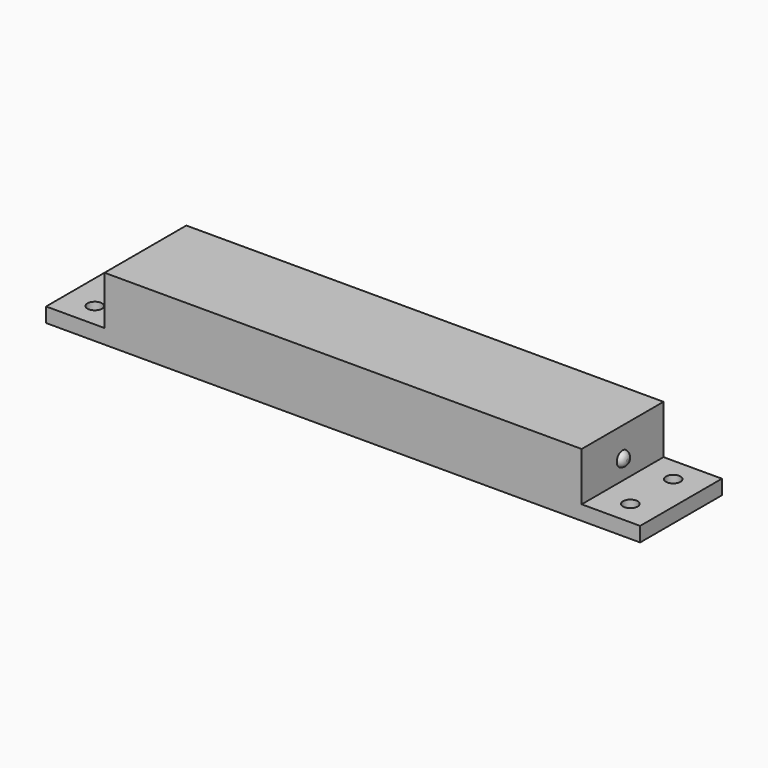
from build123d import *

# Parameters (mm, degrees)
F0_W     = 155.575
F0_H     = 33.3375
F1_DEPTH = 20.6375
F0_W_2   = 19.05
F0_R     = 2.38125
F2_DEPTH = 1.5875
F3_SIZE  = 1.27
F4_R     = 2.38125
F5_DEPTH = 1.5875
F7_DEPTH = 3.175


# Not quite as in the source:
# - a fillet or chamfer that OpenCascade refuses, or shapes differently, is made with other operations: its cross-section is extruded or revolved along the edge and cut away or added


with BuildPart() as f1:
    # F0 (on Top) → F1 (new body)
    with BuildSketch(Plane.XY):
        Rectangle(F0_W, F0_H)
    extrude(amount=F1_DEPTH)

    # F0 (on Top) → F2 (join)
    with BuildSketch(Plane.XY):
        with Locations((-87.3125, 0)):
            Rectangle(F0_W_2, F0_H)
        with Locations((-87.3125, -8.73125)):
            Circle(F0_R, mode=Mode.SUBTRACT)
        with Locations((-87.3125, 8.73125)):
            Circle(F0_R, mode=Mode.SUBTRACT)
        with Locations((87.3125, 0)):
            Rectangle(F0_W_2, F0_H)
        with Locations((87.3125, -8.73125)):
            Circle(F0_R, mode=Mode.SUBTRACT)
        with Locations((87.3125, 8.73125)):
            Circle(F0_R, mode=Mode.SUBTRACT)
    extrude(amount=F2_DEPTH)

    # F3
    f3_edges = [f1.edges().sort_by_distance(p)[0] for p in [
        (-89.69375, -8.73125, 0),
        (-89.69375, 8.73125, 0),
        (84.93125, -8.73125, 0),
        (84.93125, 8.73125, 0),
    ]]
    chamfer(f3_edges, length=F3_SIZE)

    # F4 (on face) → F5 (join)
    with BuildSketch(Plane.YZ.offset(77.7875)):
        with Locations((0, 11.1125)):
            Circle(F4_R)
    extrude(amount=F5_DEPTH)

    # F6: fillet of radius 2.032 on 1 edges, made by hand

    # F6_s1 → F6_t2 (revolve, cut)
    with BuildSketch(Plane.XY.offset(11.1125)):
        with BuildLine():
            ThreePointArc((77.7875, 2.38125), (78.9292294916, 1.6684631355), (79.375, 0.3984631355))
            Line((79.375, 0.3984631355), (79.375, 2.38125))
            Line((79.375, 2.38125), (77.7875, 2.38125))
        make_face()
    revolve(axis=Axis((79.375, 0, 11.1125), (1, 0, 0)), mode=Mode.SUBTRACT)

    # F7 (add): faces of the model
    f7_faces = [f1.faces().sort_by_distance(p)[0] for p in [
        (-87.3125, 0, 1.5875),
        (87.3125, 0, 1.5875),
    ]]
    extrude(f7_faces, amount=F7_DEPTH)


solid = f1.part
